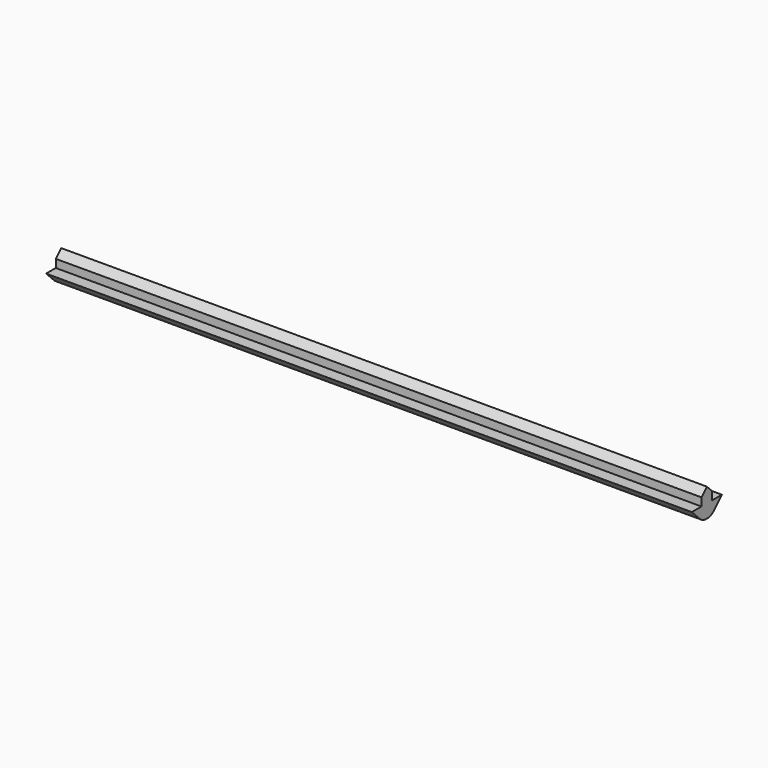
from build123d import *

# Parameters (mm, degrees)
F0_W        = 76.2
F0_H        = 1.5875
F0_H_2      = 2.38125
F1_DEPTH    = 1.5875
F2_DEPTH    = 3.81
F3_T1_DEPTH = 82.7320747894
F4_T1_DEPTH = 89.2641495789
F5_R        = 1.397


# Not quite as in the source:
# - a fillet or chamfer that OpenCascade refuses, or shapes differently, is made with other operations: its cross-section is extruded or revolved along the edge and cut away or added


with BuildPart() as f1:
    # F0 (on Top) → F1 (new body)
    with BuildSketch(Plane.XY):
        Rectangle(F0_W, F0_H)
        with Locations((0, -1.984375)):
            Rectangle(F0_W, F0_H_2)
        with Locations((0, 1.984375)):
            Rectangle(F0_W, F0_H_2)
    extrude(amount=F1_DEPTH)

    # F0 (on Top) → F2 (join)
    with BuildSketch(Plane.XY):
        Rectangle(F0_W, F0_H)
    extrude(amount=F2_DEPTH)

    # F3: chamfer of 1.27 on 2 edges, made by hand

    # F3_s2 → F3_t1 (cut)
    with BuildSketch(Plane.YZ.offset(-41.3660373947)):
        Polygon((-0.79375, 2.54), (0.47625, 3.81), (-0.79375, 3.81), align=None)
        Polygon((-0.47625, 3.81), (0.79375, 2.54), (0.79375, 3.81), align=None)
    extrude(amount=F3_T1_DEPTH, mode=Mode.SUBTRACT)

    # F4: chamfer of 2.54 on 2 edges, made by hand

    # F4_s2 → F4_t1 (cut)
    with BuildSketch(Plane.YZ.offset(-44.6320747894)):
        Polygon((-3.175, 2.54), (-0.635, 0), (-3.175, 0), align=None)
        Polygon((0.635, 0), (3.175, 2.54), (3.175, 0), align=None)
    extrude(amount=F4_T1_DEPTH, mode=Mode.SUBTRACT)

    # F5
    f5_edges = [f1.edges().sort_by_distance(p)[0] for p in [
        (0, -0.635, 0),
        (0, 0.635, 0),
    ]]
    fillet(f5_edges, radius=F5_R)


solid = f1.part
